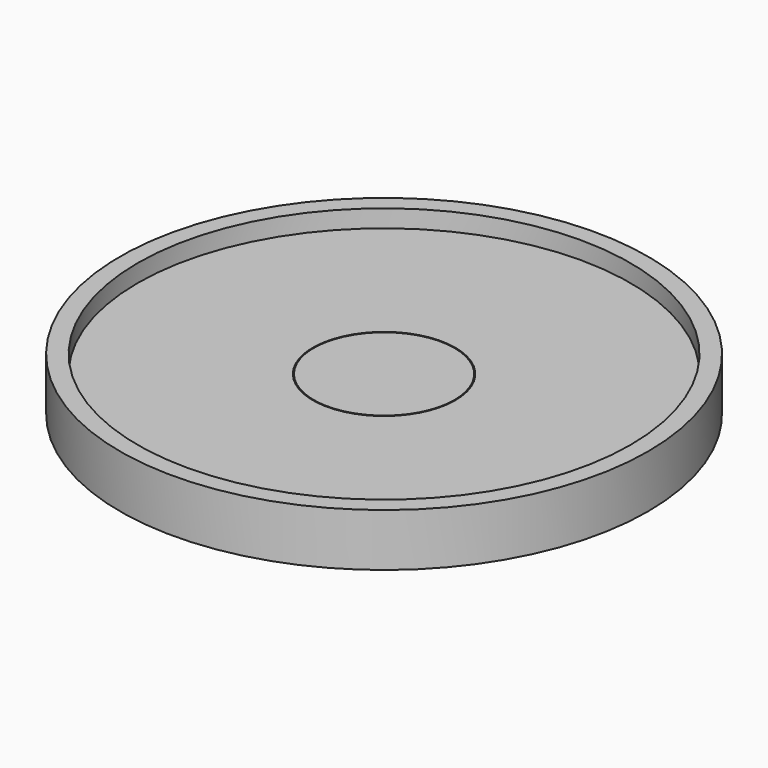
from build123d import *

# Parameters (mm, degrees)
F0_R     = 4
F1_DEPTH = 4
F0_R_2   = 4.05
F2_DEPTH = 1
F3_DEPTH = 2
F0_R_3   = 15
F0_R_4   = 14
F0_R_5   = 11
F4_DEPTH = 3


with BuildPart() as f1:
    # F0 (on Top) → F1 (new body)
    with BuildSketch(Plane.XY):
        Circle(F0_R)
    extrude(amount=-F1_DEPTH)

    # F0 (on Top) → F3 (join)
    with BuildSketch(Plane.XY):
        Circle(F0_R)
    extrude(amount=F3_DEPTH)


with BuildPart() as f2:
    # F0 (on Top) → F2 (new body)
    with BuildSketch(Plane.XY):
        Circle(F0_R_2)
        Circle(F0_R, mode=Mode.SUBTRACT)
    extrude(amount=-F2_DEPTH)


with BuildPart() as f3:
    # F0 (on Top) → F3, piece 2 (new body)
    with BuildSketch(Plane.XY):
        Circle(F0_R_3)
        Circle(F0_R_4, mode=Mode.SUBTRACT)
        Circle(F0_R_4)
        Circle(F0_R_5, mode=Mode.SUBTRACT)
        Circle(F0_R_5)
        Circle(F0_R_2, mode=Mode.SUBTRACT)
    extrude(amount=F3_DEPTH)

    # F0 (on Top) → F4 (join)
    with BuildSketch(Plane.XY):
        Circle(F0_R_3)
        Circle(F0_R_4, mode=Mode.SUBTRACT)
    extrude(amount=F4_DEPTH)


solid = Compound([f1.part, f2.part, f3.part])
